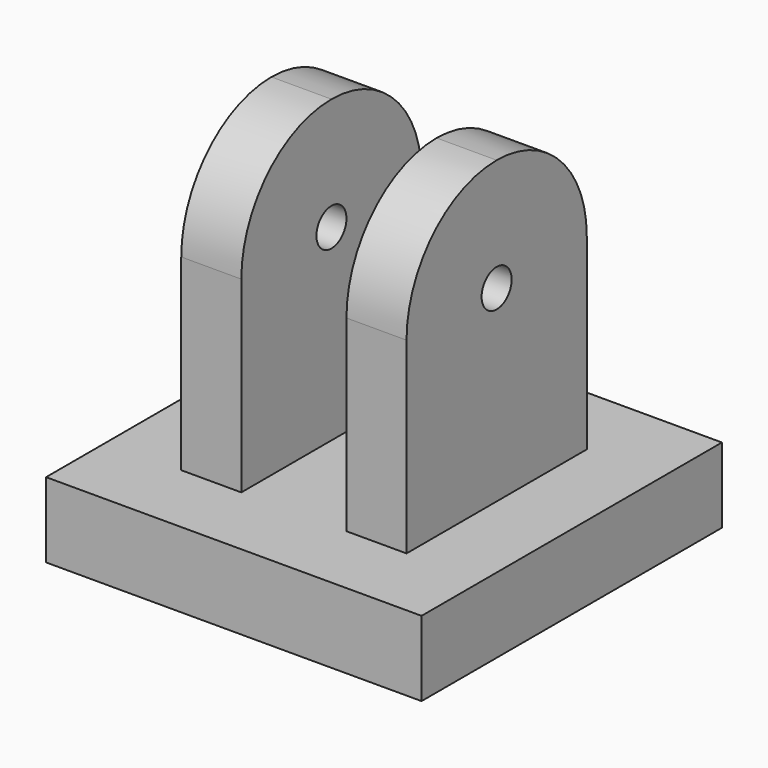
from build123d import *

# Parameters (mm, degrees)
F0_W     = 50
F0_H     = 50
F1_DEPTH = 10
F2_W     = 8
F2_H     = 30
F3_DEPTH = 40
F4_R     = 14.99999
F6_D     = 5


# Not quite as in the source:
# - a fillet or chamfer is up to 0.001 mm smaller than in the source, because OpenCascade refuses the exact size


with BuildPart() as f1:
    # F0 (on Top) → F1 (new body)
    with BuildSketch(Plane.XY):
        with Locations((3.7194620818, 6.6150704944)):
            Rectangle(F0_W, F0_H)
    extrude(amount=F1_DEPTH)

    # F2 (on face) → F3 (join)
    with BuildSketch(Plane.XY.offset(10)):
        with Locations((-7.2805379182, 6.6150704944)):
            Rectangle(F2_W, F2_H)
        with Locations((14.7194620818, 6.6150704944)):
            Rectangle(F2_W, F2_H)
    extrude(amount=F3_DEPTH)

    # F4 (radius 15 in the source; OpenCascade refuses exactly that, so slightly less here)
    f4_edges = [f1.edges().sort_by_distance(p)[0] for p in [
        (-7.280538, -8.38493, 50),
        (-7.280538, 21.61507, 50),
        (14.719462, -8.38493, 50),
        (14.719462, 21.61507, 50),
    ]]
    fillet(f4_edges, radius=F4_R)

    # F6 (through all)
    with Locations(Plane.YZ.offset(18.7194620818)):
        with Locations((6.6150704944, 35)):
            Hole(F6_D / 2)


solid = f1.part
